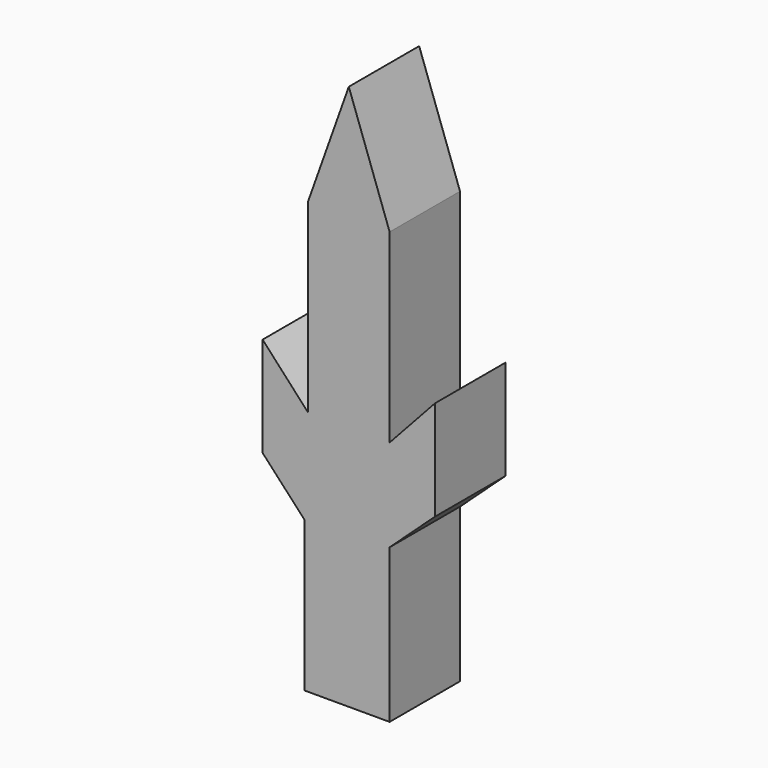
from build123d import *

# Parameters (mm, degrees)
F1_DEPTH = 25.4
F3_DEPTH = 25.4


# Not quite as in the source:
# - a feature names something its author has since deleted; it is built from what else it names


with BuildPart() as f1:
    # F0 (on Front) → F1 (new body)
    with BuildSketch(Plane.XZ):
        Polygon((11.7880795151, 53.5375215113), (0, 86.6096317768), (-11.7820905356, 53.5432), (-11.7820905356, 0), (-24.8799551113, 14.2439296469), (-24.8799551113, -14.5713714883), (-12.7764736156, -27.6303915451), (-12.7764736156, -39.4159915451), (11.7880795151, -39.4159915451), (11.7880795151, -26.6211631082), (24.8922296689, -14.5713714883), (24.8922296689, 14.2439296469), (11.7880795151, 0), align=None)
    extrude(amount=F1_DEPTH)

    # F2 (on face) → F3 (join)
    with BuildSketch(Plane.XZ.offset(25.4)):
        Polygon((-0.4971447281, -47.3129446821), (-12.7764736156, -55.2061082793), (-0.4912507866, -63.1106432249), (11.7880795151, -55.2136891784), align=None)
        Polygon((11.7880795151, -39.4159915451), (-12.7764736156, -39.4159915451), (-0.4971447281, -47.3129446821), align=None)
        Polygon((-0.4912507866, -63.1106432249), (-12.7764736156, -71.0113868117), (11.7880795151, -71.0113868117), align=None)
        Polygon((11.7880795151, -39.4159915451), (-0.4971447281, -47.3129446821), (11.7880795151, -55.2136891784), align=None)
        Polygon((-0.4971447281, -47.3129446821), (-12.7764736156, -39.4159915451), (-12.7764736156, -55.2061082793), align=None)
        Polygon((11.7880795151, -55.2136891784), (-0.4912507866, -63.1106432249), (11.7880795151, -71.0113868117), align=None)
        Polygon((-0.4912507866, -63.1106432249), (-12.7764736156, -55.2061082793), (-12.7764736156, -71.0113868117), align=None)
    extrude(amount=-F3_DEPTH)


solid = f1.part
